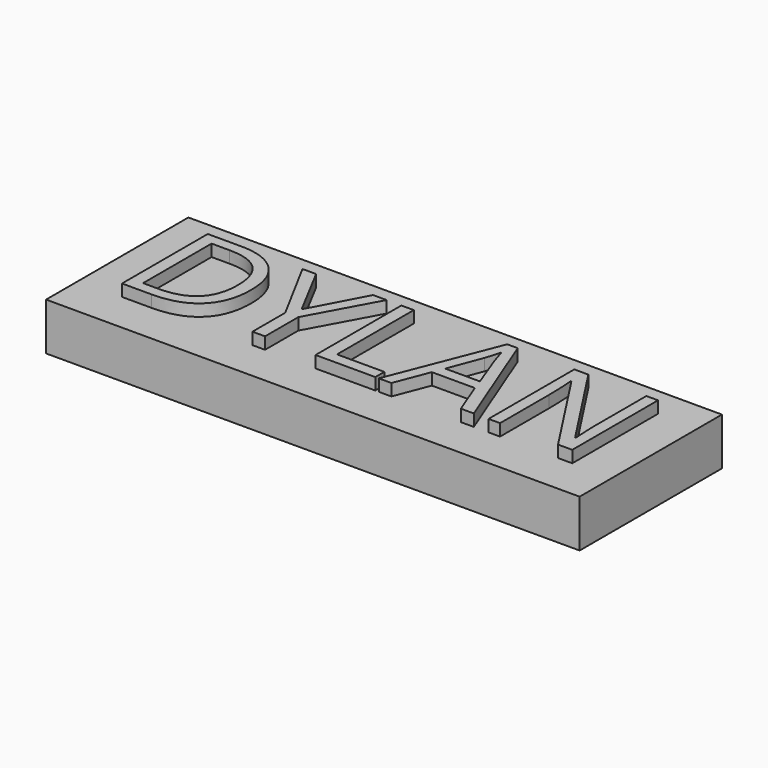
from build123d import *

# Parameters (mm, degrees)
F0_W         = 114.3
F0_H         = 38.1
F1_DEPTH     = 10.16
F0_TEXT_SIZE = 32.1677620781
F2_DEPTH     = 12.7


# Not quite as in the source:
# - Text() gives the source's letters only with a copy of the font that has no kerning and outlines rounded to 1/6400 em; it was checked with that copy


with BuildPart() as f1:
    # F0 (on Top) → F1 (new body)
    with BuildSketch(Plane.XY):
        Rectangle(F0_W, F0_H)
        with BuildLine():
            add(Edge.make_bspline(
                [(-32.4647352326, 9.6195506155), (-29.4967565596, 6.6515719425), (-29.4967565596, 1.3237863483)],
                knots=[0, 0, 0, 1, 1, 1], degree=2))
            add(Edge.make_bspline(
                [(-29.4967565596, 1.3237863483), (-29.4967565596, -4.3608603564), (-32.582851234, -7.369048732)],
                knots=[0, 0, 0, 1, 1, 1], degree=2))
            add(Edge.make_bspline(
                [(-32.582851234, -7.369048732), (-35.6689459084, -10.3772371076), (-41.4641692953, -10.3772371076)],
                knots=[0, 0, 0, 1, 1, 1], degree=2))
            Line((-41.4641692953, -10.3772371076), (-47.8273547314, -10.3772371076))
            Line((-47.8273547314, -10.3772371076), (-47.8273547314, 12.5875292885))
            Line((-47.8273547314, 12.5875292885), (-40.7906567768, 12.5875292885))
            add(Edge.make_bspline(
                [(-40.7906567768, 12.5875292885), (-35.4327139056, 12.5875292885), (-32.4647352326, 9.6195506155)],
                knots=[0, 0, 0, 1, 1, 1], degree=2))
        make_face(mode=Mode.SUBTRACT)
        Polygon((-24.611277694, 12.5875292885), (-18.5295601761, 1.102632984), (-12.4076329556, 12.5875292885), (-9.5175605814, 12.5875292885), (-17.1825351391, -1.4707879822), (-17.1825351391, -10.3772371076), (-19.881611426, -10.3772371076), (-19.881611426, -1.5964433028), (-27.5315073452, 12.5875292885), align=None, mode=Mode.SUBTRACT)
        Polygon((6.440665137, -10.3772371076), (-6.3610989275, -10.3772371076), (-6.3610989275, 12.5875292885), (-3.6921799176, 12.5875292885), (-3.6921799176, -7.9596287389), (6.440665137, -7.9596287389), align=None, mode=Mode.SUBTRACT)
        Polygon((27.5356803623, -10.3772371076), (24.7712633087, -10.3772371076), (21.9113482115, -3.0741498733), (12.7083525294, -3.0741498733), (9.883620922, -10.3772371076), (7.1795184223, -10.3772371076), (16.2568587837, 12.6830273322), (18.5035759163, 12.6830273322), align=None, mode=Mode.SUBTRACT)
        with BuildLine():
            Line((48.6306955876, 12.5875292885), (48.6306955876, -10.3772371076))
            Line((48.6306955876, -10.3772371076), (45.5848106159, -10.3772371076))
            Line((45.5848106159, -10.3772371076), (33.0343571926, 8.8932628623))
            Line((33.0343571926, 8.8932628623), (32.9087018719, 8.8932628623))
            add(Edge.make_bspline(
                [(32.9087018719, 8.8932628623), (33.1600125132, 5.5005692057), (33.1600125132, 2.6758375982)],
                knots=[0, 0, 0, 1, 1, 1], degree=2))
            Line((33.1600125132, 2.6758375982), (33.1600125132, -10.3772371076))
            Line((33.1600125132, -10.3772371076), (30.6921420163, -10.3772371076))
            Line((30.6921420163, -10.3772371076), (30.6921420163, 12.5875292885))
            Line((30.6921420163, 12.5875292885), (33.7078697111, 12.5875292885))
            Line((33.7078697111, 12.5875292885), (46.2281658574, -6.6075774891))
            Line((46.2281658574, -6.6075774891), (46.353821178, -6.6075774891))
            add(Edge.make_bspline(
                [(46.353821178, -6.6075774891), (46.3236639011, -6.1853756118), (46.213087219, -3.8833701381)],
                knots=[0, 0, 0, 1, 1, 1], degree=2))
            add(Edge.make_bspline(
                [(46.213087219, -3.8833701381), (46.1025105368, -1.5813646644), (46.1326678138, -0.5912007379)],
                knots=[0, 0, 0, 1, 1, 1], degree=2))
            Line((46.1326678138, -0.5912007379), (46.1326678138, 12.5875292885))
            Line((46.1326678138, 12.5875292885), (48.6306955876, 12.5875292885))
        make_face(mode=Mode.SUBTRACT)
    extrude(amount=F1_DEPTH)



with BuildPart() as f1b:
    # F0 (on Top) → F1, piece 2 (new body)
    with BuildSketch(Plane.XY):
        with BuildLine():
            add(Edge.make_bspline(
                [(-34.7265310037, -5.7204509255), (-32.3214881671, -3.37069643), (-32.3214881671, 1.2282883046)],
                knots=[0, 0, 0, 1, 1, 1], degree=2))
            add(Edge.make_bspline(
                [(-32.3214881671, 1.2282883046), (-32.3214881671, 5.7217225699), (-34.575744619, 7.9985969795)],
                knots=[0, 0, 0, 1, 1, 1], degree=2))
            add(Edge.make_bspline(
                [(-34.575744619, 7.9985969795), (-36.8300010709, 10.2754713891), (-41.2781994208, 10.2754713891)],
                knots=[0, 0, 0, 1, 1, 1], degree=2))
            Line((-41.2781994208, 10.2754713891), (-45.1584357214, 10.2754713891))
            Line((-45.1584357214, 10.2754713891), (-45.1584357214, -8.0702054211))
            Line((-45.1584357214, -8.0702054211), (-41.9064760238, -8.0702054211))
            add(Edge.make_bspline(
                [(-41.9064760238, -8.0702054211), (-37.1315738404, -8.0702054211), (-34.7265310037, -5.7204509255)],
                knots=[0, 0, 0, 1, 1, 1], degree=2))
        make_face()
    extrude(amount=F1_DEPTH)


with BuildPart() as f1c:
    # F0 (on Top) → F1, piece 3 (new body)
    with BuildSketch(Plane.XY):
        with BuildLine():
            Line((13.6532805405, -0.6716201431), (21.0820230954, -0.6716201431))
            Line((21.0820230954, -0.6716201431), (18.4080778727, 6.4454972167))
            add(Edge.make_bspline(
                [(18.4080778727, 6.4454972167), (17.8903779517, 7.7975484665), (17.3425207538, 9.7577714682)],
                knots=[0, 0, 0, 1, 1, 1], degree=2))
            add(Edge.make_bspline(
                [(17.3425207538, 9.7577714682), (16.9957120689, 8.2499076208), (16.3523568274, 6.4454972167)],
                knots=[0, 0, 0, 1, 1, 1], degree=2))
            Line((16.3523568274, 6.4454972167), (13.6532805405, -0.6716201431))
        make_face()
    extrude(amount=F1_DEPTH)


with BuildPart() as f1_1:
    add(f1.part)

    add(f1b.part)  # F2 merges F1b

    add(f1c.part)  # F2 merges F1c
    # F0 (on Top) → F2 (join)
    with BuildSketch(Plane.XY):
        with Locations((-50.9838163853, -10.3772371076)):
            Text('DYLAN', F0_TEXT_SIZE, font='Open Sans', text_align=(TextAlign.LEFT, TextAlign.BOTTOM))
    extrude(amount=F2_DEPTH)


solid = f1_1.part
